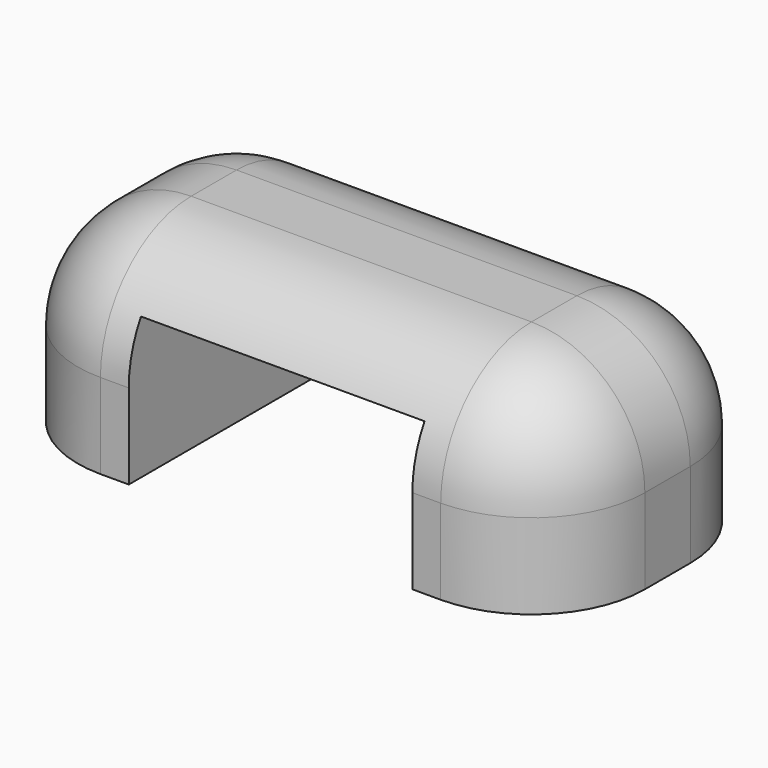
from build123d import *

# Parameters (mm, degrees)
F0_W         = 5
F0_H         = 10
F1_DEPTH     = 5
F2_W         = 20
F2_H         = 10
F3_DEPTH     = 2
F4_T1_DEPTH  = 2
F4_T3_DEPTH  = 12
F4_T5_DEPTH  = 13
F4_S9_W      = 4
F4_S9_H      = 4
F4_T10_DEPTH = 4
F4_S15_W     = 4
F4_S15_H     = 4
F4_T16_DEPTH = 4
F4_S21_W     = 4
F4_S21_H     = 4
F4_T22_DEPTH = 4
F4_S27_W     = 4
F4_S27_H     = 4
F4_T28_DEPTH = 4


# Not quite as in the source:
# - a fillet or chamfer that OpenCascade refuses, or shapes differently, is made with other operations: its cross-section is extruded or revolved along the edge and cut away or added


with BuildPart() as f1:
    # F0 (on Top) → F1 (new body)
    with BuildSketch(Plane.XY):
        with Locations((-7.5, 0)):
            Rectangle(F0_W, F0_H)
    extrude(amount=F1_DEPTH)



with BuildPart() as f1b:
    # F0 (on Top) → F1, piece 2 (new body)
    with BuildSketch(Plane.XY):
        with Locations((7.5, 0)):
            Rectangle(F0_W, F0_H)
    extrude(amount=F1_DEPTH)


with BuildPart() as f1_1:
    add(f1.part)

    add(f1b.part)  # F3 merges F1b
    # F2 (on face) → F3 (join)
    with BuildSketch(Plane.XY.offset(5)):
        Rectangle(F2_W, F2_H)
    extrude(amount=F3_DEPTH)

    # F4: fillet of radius 4 on 8 edges, made by hand

    # F4_s2 → F4_t1 (cut)
    with BuildSketch(Plane.XZ.offset(-1)):
        with BuildLine():
            ThreePointArc((-10, 3), (-8.8284271247, 5.8284271247), (-6, 7))
            Line((-6, 7), (-10, 7))
            Line((-10, 7), (-10, 3))
        make_face()
        with BuildLine():
            ThreePointArc((6, 7), (8.8284271247, 5.8284271247), (10, 3))
            Line((10, 3), (10, 7))
            Line((10, 7), (6, 7))
        make_face()
    extrude(amount=F4_T1_DEPTH, mode=Mode.SUBTRACT)

    # F4_s4 → F4_t3 (cut)
    with BuildSketch(Plane.YZ.offset(-6)):
        with BuildLine():
            ThreePointArc((-5, 3), (-3.8284271247, 5.8284271247), (-1, 7))
            Line((-1, 7), (-5, 7))
            Line((-5, 7), (-5, 3))
        make_face()
        with BuildLine():
            ThreePointArc((5, 3), (3.8284271247, 5.8284271247), (1, 7))
            Line((1, 7), (5, 7))
            Line((5, 7), (5, 3))
        make_face()
    extrude(amount=F4_T3_DEPTH, mode=Mode.SUBTRACT)

    # F4_s6 → F4_t5 (cut)
    with BuildSketch(Plane.XY.offset(-10)):
        with BuildLine():
            ThreePointArc((6, -5), (8.8284271247, -3.8284271247), (10, -1))
            Line((10, -1), (10, -5))
            Line((10, -5), (6, -5))
        make_face()
        with BuildLine():
            ThreePointArc((6, 5), (8.8284271247, 3.8284271247), (10, 1))
            Line((10, 1), (10, 5))
            Line((10, 5), (6, 5))
        make_face()
        with BuildLine():
            ThreePointArc((-6, 5), (-8.8284271247, 3.8284271247), (-10, 1))
            Line((-10, 1), (-10, 5))
            Line((-10, 5), (-6, 5))
        make_face()
        with BuildLine():
            ThreePointArc((-6, -5), (-8.8284271247, -3.8284271247), (-10, -1))
            Line((-10, -1), (-10, -5))
            Line((-10, -5), (-6, -5))
        make_face()
    extrude(amount=F4_T5_DEPTH, mode=Mode.SUBTRACT)


with BuildPart() as f4_tool8:
    # F4_s9 → F4_t10 (new body)
    with BuildSketch(Plane.XY.offset(3)):
        with Locations((-8, 3)):
            Rectangle(F4_S9_W, F4_S9_H)
    extrude(amount=F4_T10_DEPTH)

    # F4_s11 → F4_t12 (revolve, cut)
    with BuildSketch(Plane(origin=(-6, 1, 3), x_dir=(0.7071067812, -0.7071067812, 0), z_dir=(-0.7071067812, -0.7071067812, 0))):
        with BuildLine():
            ThreePointArc((0, -4), (4, 0), (0, 4))
            Line((0, 4), (0, -4))
        make_face()
    revolve(axis=Axis((-6, 1, 3), (0, 0, 1)), mode=Mode.SUBTRACT)


with BuildPart() as f1_2:
    add(f1_1.part)

    # F4_t7: cut F4_tool8
    add(f4_tool8.part, mode=Mode.SUBTRACT)


with BuildPart() as f4_tool14:
    # F4_s15 → F4_t16 (new body)
    with BuildSketch(Plane.XY.offset(3)):
        with Locations((-8, -3)):
            Rectangle(F4_S15_W, F4_S15_H)
    extrude(amount=F4_T16_DEPTH)

    # F4_s17 → F4_t18 (revolve, cut)
    with BuildSketch(Plane(origin=(-6, -1, 3), x_dir=(0.7071067812, 0.7071067812, 0), z_dir=(0.7071067812, -0.7071067812, 0))):
        with BuildLine():
            ThreePointArc((0, -4), (4, 0), (0, 4))
            Line((0, 4), (0, -4))
        make_face()
    revolve(axis=Axis((-6, -1, 3), (0, 0, 1)), mode=Mode.SUBTRACT)


with BuildPart() as f1_3:
    add(f1_2.part)

    # F4_t13: cut F4_tool14
    add(f4_tool14.part, mode=Mode.SUBTRACT)


with BuildPart() as f4_tool20:
    # F4_s21 → F4_t22 (new body)
    with BuildSketch(Plane.XY.offset(3)):
        with Locations((8, -3)):
            Rectangle(F4_S21_W, F4_S21_H)
    extrude(amount=F4_T22_DEPTH)

    # F4_s23 → F4_t24 (revolve, cut)
    with BuildSketch(Plane(origin=(6, -1, 3), x_dir=(-0.7071067812, 0.7071067812, 0), z_dir=(0.7071067812, 0.7071067812, 0))):
        with BuildLine():
            ThreePointArc((0, -4), (4, 0), (0, 4))
            Line((0, 4), (0, -4))
        make_face()
    revolve(axis=Axis((6, -1, 3), (0, 0, 1)), mode=Mode.SUBTRACT)


with BuildPart() as f1_4:
    add(f1_3.part)

    # F4_t19: cut F4_tool20
    add(f4_tool20.part, mode=Mode.SUBTRACT)


with BuildPart() as f4_tool26:
    # F4_s27 → F4_t28 (new body)
    with BuildSketch(Plane.XY.offset(3)):
        with Locations((8, 3)):
            Rectangle(F4_S27_W, F4_S27_H)
    extrude(amount=F4_T28_DEPTH)

    # F4_s29 → F4_t30 (revolve, cut)
    with BuildSketch(Plane(origin=(6, 1, 3), x_dir=(-0.7071067812, -0.7071067812, 0), z_dir=(-0.7071067812, 0.7071067812, 0))):
        with BuildLine():
            ThreePointArc((0, -4), (4, 0), (0, 4))
            Line((0, 4), (0, -4))
        make_face()
    revolve(axis=Axis((6, 1, 3), (0, 0, 1)), mode=Mode.SUBTRACT)


with BuildPart() as f1_5:
    add(f1_4.part)

    # F4_t25: cut F4_tool26
    add(f4_tool26.part, mode=Mode.SUBTRACT)


solid = f1_5.part
